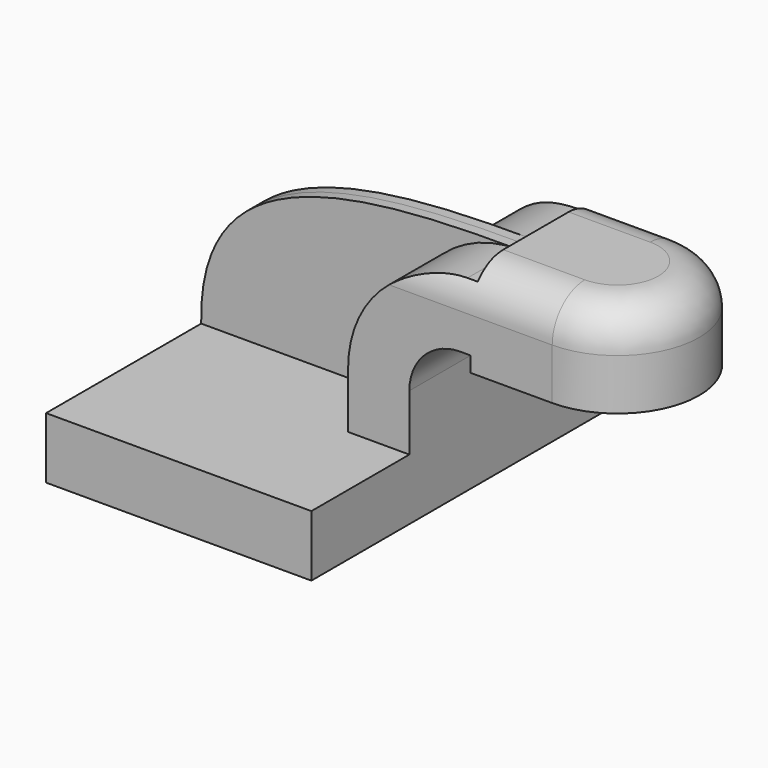
from build123d import *

# Parameters (mm, degrees)
F1_DEPTH = 63.5
F0_W     = 25.4
F0_H     = 19.05
F0_H_2   = 4.7752
F0_H_3   = 4.7498
F2_DEPTH = 25.4
F4_DEPTH = 3.175
F5_R     = 12.7


with BuildPart() as f1:
    # F0 (on Front) → F1 (new body, symmetric)
    with BuildSketch(Plane.XZ):
        Polygon((-41.275, -9.525), (41.275, -9.525), (41.275, 9.525), (22.225, 9.525), (-41.275, 9.525), align=None)
    extrude(amount=F1_DEPTH, both=True)

    # F0 (on Front) → F2 (join, symmetric)
    with BuildSketch(Plane.XZ):
        with BuildLine():
            Line((22.225, 9.525), (41.275, 9.525))
            Line((41.275, 9.525), (41.275, 27.0002))
            ThreePointArc((41.275, 27.0002), (45.9246798487, 38.2255201513), (57.15, 42.8752))
            Line((57.15, 42.8752), (60.325, 42.8752))
            Line((60.325, 42.8752), (60.325, 61.9252))
            Line((60.325, 61.9252), (57.15, 61.9252))
            ThreePointArc((57.15, 61.9252), (32.4542956671, 51.6959043329), (22.225, 27.0002))
            Line((22.225, 27.0002), (22.225, 9.525))
        make_face()
        with Locations((73.025, 52.4002)):
            Rectangle(F0_W, F0_H)
        with Locations((73.025, 40.4876)):
            Rectangle(F0_W, F0_H_2)
        with Locations((73.025, 64.3001)):
            Rectangle(F0_W, F0_H_3)
    extrude(amount=F2_DEPTH, both=True)

    # F0 (on Front) → F3 (revolve)
    with BuildSketch(Plane.XZ):
        Polygon((85.725, 66.675), (85.725, 61.9252), (85.725, 42.8752), (85.725, 38.1), (111.125, 38.1), (111.125, 66.675), align=None)
    revolve(axis=Axis((85.725, 0, 52.3875), (0, 0, 1)))

    # F0 (on Front) → F4 (join, symmetric)
    with BuildSketch(Plane.XZ):
        with BuildLine():
            add(Edge.make_bspline(
                [(-41.275, 9.525), (-42.3543564975, 56.6976591945), (4.171225708, 62.171254307), (57.15, 61.9252)],
                knots=[0, 0, 0, 0, 111.5045361635, 111.5045361635, 111.5045361635, 111.5045361635], degree=3))
            Line((-41.275, 9.525), (22.225, 9.525))
            Line((22.225, 9.525), (22.225, 27.0002))
            ThreePointArc((22.225, 27.0002), (32.4542956671, 51.6959043329), (57.15, 61.9252))
        make_face()
    extrude(amount=F4_DEPTH, both=True)

    # F5
    f5_edges = [f1.edges().sort_by_distance(p)[0] for p in [
        (85.725, 25.4, 52.3875),
        (73.025, 25.4, 66.675),
        (73.025, -25.4, 66.675),
        (111.125, 0, 66.675),
    ]]
    fillet(f5_edges, radius=F5_R)


solid = f1.part
